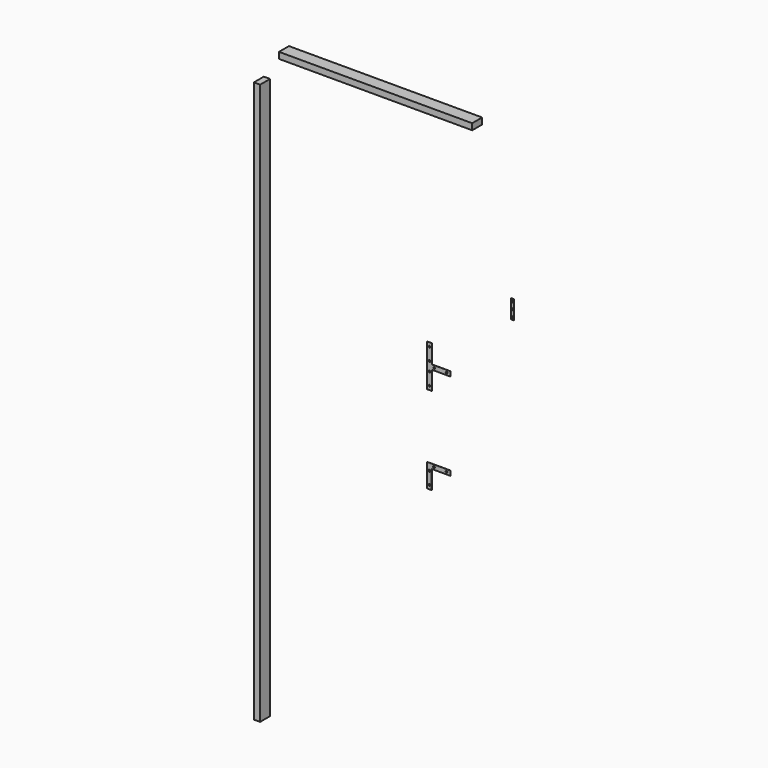
from build123d import *

# Parameters (mm, degrees)
F1_W      = 787.4
F1_H      = 25.4
F2_DEPTH  = 50.8
F0_W      = 25.4
F0_H      = 2286
F3_DEPTH  = 50.8
F4_R      = 3.175
F5_DEPTH  = 0.635
F6_R      = 3.175
F7_DEPTH  = 0.635
F8_SIZE   = 0.63499
F9_SIZE   = 0.63499
F10_W     = 12.7
F10_H     = 76.2
F10_R     = 3.175
F11_DEPTH = 0.635
F12_SIZE  = 0.63499


# Not quite as in the source:
# - a fillet or chamfer is up to 0.001 mm smaller than in the source, because OpenCascade refuses the exact size


with BuildPart() as f2:
    # F1 (on Front) → F2 (new body)
    with BuildSketch(Plane.XZ):
        with Locations((455.4581004176, 2289.2231941223)):
            Rectangle(F1_W, F1_H)
    extrude(amount=F2_DEPTH)


with BuildPart() as f3:
    # F0 (on Front) → F3 (new body)
    with BuildSketch(Plane.XZ):
        with Locations((-27.7979671955, 1016.1481191226)):
            Rectangle(F0_W, F0_H)
    extrude(amount=F3_DEPTH)


with BuildPart() as f5:
    # F4 (on Front) → F5 (new body)
    with BuildSketch(Plane.XZ):
        Polygon((624.6407955857, 993.5723245871), (624.6407955857, 898.3223245871), (643.6907955857, 898.3223245871), (643.6907955857, 974.5223245871), (719.8907955857, 974.5223245871), (719.8907955857, 993.5723245871), align=None)
        with Locations((634.1657955857, 914.1973245871)):
            Circle(F4_R, mode=Mode.SUBTRACT)
        with Locations((634.1657955857, 964.9973245871)):
            Circle(F4_R, mode=Mode.SUBTRACT)
        with Locations((653.2157955857, 984.0473245871)):
            Circle(F4_R, mode=Mode.SUBTRACT)
        with Locations((704.0157955857, 984.0473245871)):
            Circle(F4_R, mode=Mode.SUBTRACT)
    extrude(amount=F5_DEPTH)

    # F9 (size 0.635 in the source; OpenCascade refuses exactly that, so slightly less here)
    f9_edges = [f5.edges().sort_by_distance(p)[0] for p in [
        (700.840796, -0.635, 984.047325),
        (650.040796, -0.635, 984.047325),
        (630.990796, -0.635, 964.997325),
        (630.990796, -0.635, 914.197325),
    ]]
    chamfer(f9_edges, length=F9_SIZE)


with BuildPart() as f7:
    # F6 (on Front) → F7 (new body)
    with BuildSketch(Plane.XZ):
        Polygon((625.4843616006, 1425.8529662132), (625.4843616006, 1254.4029662132), (644.5343616006, 1254.4029662132), (644.5343616006, 1330.6029662132), (720.7343616006, 1330.6029662132), (720.7343616006, 1349.6529662132), (644.5343616006, 1349.6529662132), (644.5343616006, 1425.8529662132), align=None)
        with Locations((635.0093616006, 1270.2779662132)):
            Circle(F6_R, mode=Mode.SUBTRACT)
        with Locations((635.0093616006, 1321.0779662132)):
            Circle(F6_R, mode=Mode.SUBTRACT)
        with Locations((654.0593616006, 1340.1279662132)):
            Circle(F6_R, mode=Mode.SUBTRACT)
        with Locations((704.8593616006, 1340.1279662132)):
            Circle(F6_R, mode=Mode.SUBTRACT)
        with Locations((635.0093616006, 1359.1779662132)):
            Circle(F6_R, mode=Mode.SUBTRACT)
        with Locations((635.0093616006, 1409.9779662132)):
            Circle(F6_R, mode=Mode.SUBTRACT)
    extrude(amount=F7_DEPTH)

    # F8 (size 0.635 in the source; OpenCascade refuses exactly that, so slightly less here)
    f8_edges = [f7.edges().sort_by_distance(p)[0] for p in [
        (701.684362, -0.635, 1340.127966),
        (650.884362, -0.635, 1340.127966),
        (631.834362, -0.635, 1321.077966),
        (631.834362, -0.635, 1270.277966),
        (631.834362, -0.635, 1359.177966),
        (631.834362, -0.635, 1409.977966),
    ]]
    chamfer(f8_edges, length=F8_SIZE)


with BuildPart() as f11:
    # F10 (on Front) → F11 (new body)
    with BuildSketch(Plane.XZ):
        with Locations((972.9659259319, 1654.346266764)):
            Rectangle(F10_W, F10_H)
        with Locations((972.9659259319, 1625.771266764)):
            Circle(F10_R, mode=Mode.SUBTRACT)
        with Locations((972.9659259319, 1654.5367240906)):
            Circle(F10_R, mode=Mode.SUBTRACT)
        with Locations((972.9659259319, 1682.921266764)):
            Circle(F10_R, mode=Mode.SUBTRACT)
    extrude(amount=F11_DEPTH)

    # F12 (size 0.635 in the source; OpenCascade refuses exactly that, so slightly less here)
    f12_edges = [f11.edges().sort_by_distance(p)[0] for p in [
        (969.790926, -0.635, 1625.771267),
        (969.790926, -0.635, 1654.536724),
        (969.790926, -0.635, 1682.921267),
    ]]
    chamfer(f12_edges, length=F12_SIZE)


solid = Compound([f2.part, f3.part, f5.part, f7.part, f11.part])
